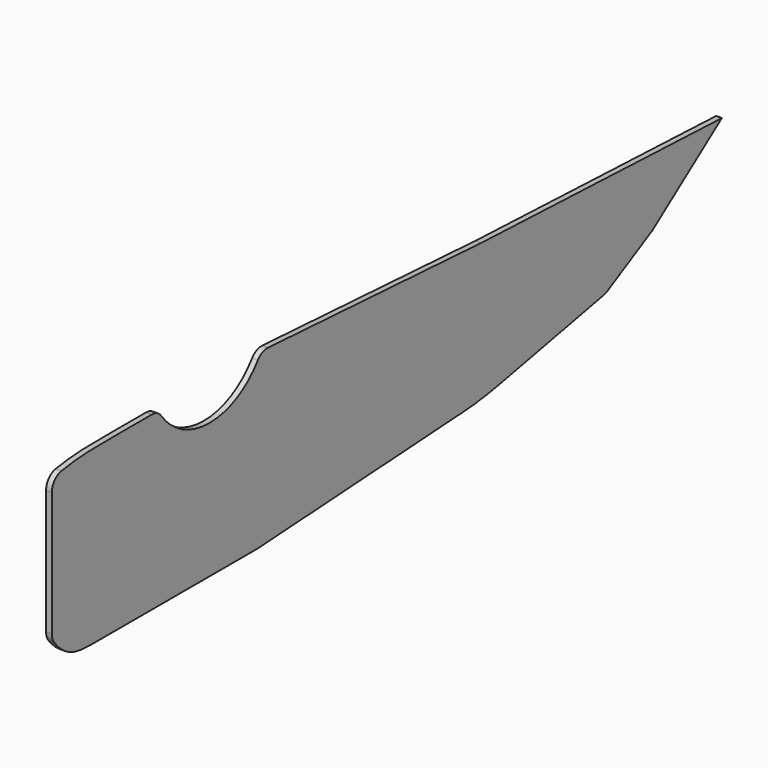
from build123d import *

# Parameters (mm, degrees)
F1_DEPTH    = 2
F2_R        = 5
F3_R        = 120.7003354098
F4_T1_DEPTH = 5.3985988059
F4_T3_DEPTH = 3.4901996791
F4_T5_DEPTH = 2.6811462233


# Not quite as in the source:
# - a fillet or chamfer that OpenCascade refuses, or shapes differently, is made with other operations: its cross-section is extruded or revolved along the edge and cut away or added
# - a feature names something its author has since deleted; it is built from what else it names


with BuildPart() as f1:
    # F0 (on Right) → F1 (new body)
    with BuildSketch(Plane.YZ):
        with BuildLine():
            add(Edge.make_bspline(
                [(-93.5, -19.165366888), (-87.3498469591, -27.7392359194), (-82.2530835867, -27.7392359194), (-74.081517756, -27.7392359194)],
                knots=[0, 0, 0, 0, 21.227074288, 21.227074288, 21.227074288, 21.227074288], degree=3))
            Line((-74.081517756, -27.7392359194), (-3.9580739103, -27.7392359194))
            Line((-3.9580739103, -27.7392359194), (93.5, -21.748252213))
            Line((93.5, -21.748252213), (147.8121578693, -11.1020449549))
            Line((147.8121578693, -11.1020449549), (168.2493239641, 0))
            Line((168.2493239641, 0), (198.5184252262, 22.1527013928))
            Line((198.5184252262, 22.1527013928), (93.5, 26.4736590703))
            Line((93.5, 26.4736590703), (-2.2493870929, 32.2607640806))
            ThreePointArc((-2.2493870929, 32.2607640806), (-24.7432854958, 19.3285844403), (-47.2371838987, 32.2607640806))
            add(Edge.make_bspline(
                [(-47.2371838987, 32.2607640806), (-62.6581225991, 31.5082555435), (-78.7113010883, 33.5351414979), (-93.5, 30.0032384694)],
                knots=[0, 0, 0, 0, 46.3178645396, 46.3178645396, 46.3178645396, 46.3178645396], degree=3))
            Line((-93.5, 30.0032384694), (-93.5, -19.165366888))
        make_face()
    extrude(amount=F1_DEPTH)

    # F2
    f2_edges = [f1.edges().sort_by_distance(p)[0] for p in [
        (1, -93.5, 30.003238),
        (1, -47.237184, 32.260764),
        (1, -2.249387, 32.260764),
        (1, -93.5, -19.165367),
        (1, -3.958074, -27.739236),
    ]]
    fillet(f2_edges, radius=F2_R)

    # F3
    f3_edges = [f1.edges().sort_by_distance(p)[0] for p in [
        (1, 93.5, -21.748252),
    ]]
    fillet(f3_edges, radius=F3_R)

    # F4: fillet of radius 4.436390167 on 3 edges, made by hand

    # F4_s2 → F4_t1 (cut)
    with BuildSketch(Plane.YZ.offset(-1.699299403)):
        with BuildLine():
            ThreePointArc((147.14513202, -11.2327946013), (147.7946205368, -11.0533364649), (148.4094389633, -10.7775850212))
            Line((148.4094389633, -10.7775850212), (147.8121578693, -11.1020449549))
            Line((147.8121578693, -11.1020449549), (147.14513202, -11.2327946013))
        make_face()
    extrude(amount=F4_T1_DEPTH, mode=Mode.SUBTRACT)

    # F4_s4 → F4_t3 (cut)
    with BuildSketch(Plane.YZ.offset(-0.7450998395)):
        with BuildLine():
            ThreePointArc((167.9874313003, -0.1422674804), (168.2439722622, 0.0084474426), (168.4898338923, 0.176019254))
            Line((168.4898338923, 0.176019254), (168.2493239641, 0))
            Line((168.2493239641, 0), (167.9874313003, -0.1422674804))
        make_face()
    extrude(amount=F4_T3_DEPTH, mode=Mode.SUBTRACT)

    # F4_s6 → F4_t5 (cut)
    with BuildSketch(Plane.YZ.offset(-0.3405731116)):
        with BuildLine():
            ThreePointArc((-3.822101334, -27.730877356), (-3.9581380925, -27.7371457861), (-4.094303155, -27.7392359194))
            Line((-4.094303155, -27.7392359194), (-3.9580739103, -27.7392359194))
            Line((-3.9580739103, -27.7392359194), (-3.822101334, -27.730877356))
        make_face()
    extrude(amount=F4_T5_DEPTH, mode=Mode.SUBTRACT)


solid = f1.part
